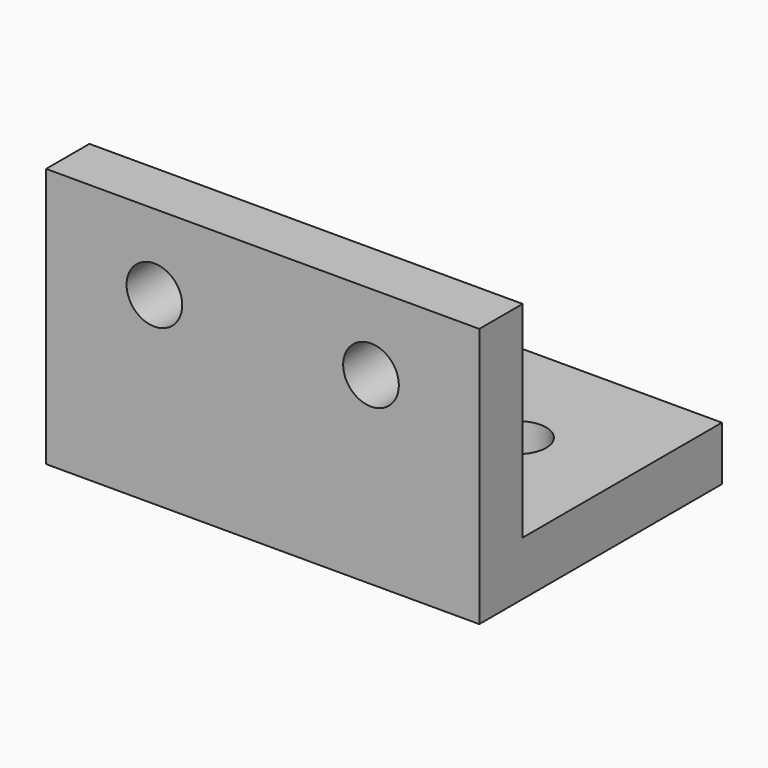
from build123d import *

# Parameters (mm, degrees)
F0_W      = 25.4
F0_H      = 3.175
F1_DEPTH  = 25.4
F2_W      = 3.175
F2_H      = 15.24
F3_DEPTH  = 25.4
F5_D      = 3.2639
F5_DEPTH  = 12.7
F5_TIP    = 0.9805744872
F7_D      = 3.2639
F7_DEPTH  = 12.7
F7_TIP    = 0.9805744872
F8_W      = 25.4
F8_H      = 3.175
F9_DEPTH  = 3.176
F11_DEPTH = 3.176


with BuildPart() as f1:
    # F0 (on Front) → F1 (new body)
    with BuildSketch(Plane.XZ):
        with Locations((13.8182396877, 1.5875)):
            Rectangle(F0_W, F0_H)
    extrude(amount=F1_DEPTH)

    # F2 (on face) → F3 (join)
    with BuildSketch(Plane.YZ.offset(26.5182396877)):
        with Locations((-23.8125, 10.795)):
            Rectangle(F2_W, F2_H)
    extrude(amount=-F3_DEPTH)

    # F5
    with Locations(Plane(origin=(0, -22.225, 0), x_dir=(-1, 0, 0), z_dir=(0, 1, 0))):
        with Locations((-20.1682396877, 10.795), (-7.4682396877, 10.795)):
            Hole(F5_D / 2, depth=F5_DEPTH)
            with Locations((0, 0, -(F5_DEPTH + F5_TIP / 2))):  # 118° drill point
                Cone(0, F5_D / 2, F5_TIP, mode=Mode.SUBTRACT)

    # F7
    with Locations(Plane.XY.offset(3.175)):
        with Locations((7.4682396877, -14.605), (20.1682396877, -14.605)):
            Hole(F7_D / 2, depth=F7_DEPTH)
            with Locations((0, 0, -(F7_DEPTH + F7_TIP / 2))):  # 118° drill point
                Cone(0, F7_D / 2, F7_TIP, mode=Mode.SUBTRACT)

    # F8 (on face) → F9 (cut, through all)
    with BuildSketch(Plane(origin=(0, -22.225, 0), x_dir=(-1, 0, 0), z_dir=(0, 1, 0))):
        with Locations((-13.8182396877, 16.8275)):
            Rectangle(F8_W, F8_H)
    extrude(amount=-F9_DEPTH, mode=Mode.SUBTRACT)

    # F10 (on face) → F11 (cut, through all)
    with BuildSketch(Plane.XY.offset(3.175)):
        Polygon((13.8182396877, 0), (1.1182396877, 0), (1.1182396877, -7.62), (26.5182396877, -7.62), (26.5182396877, 0), align=None)
    extrude(amount=-F11_DEPTH, mode=Mode.SUBTRACT)


solid = f1.part
